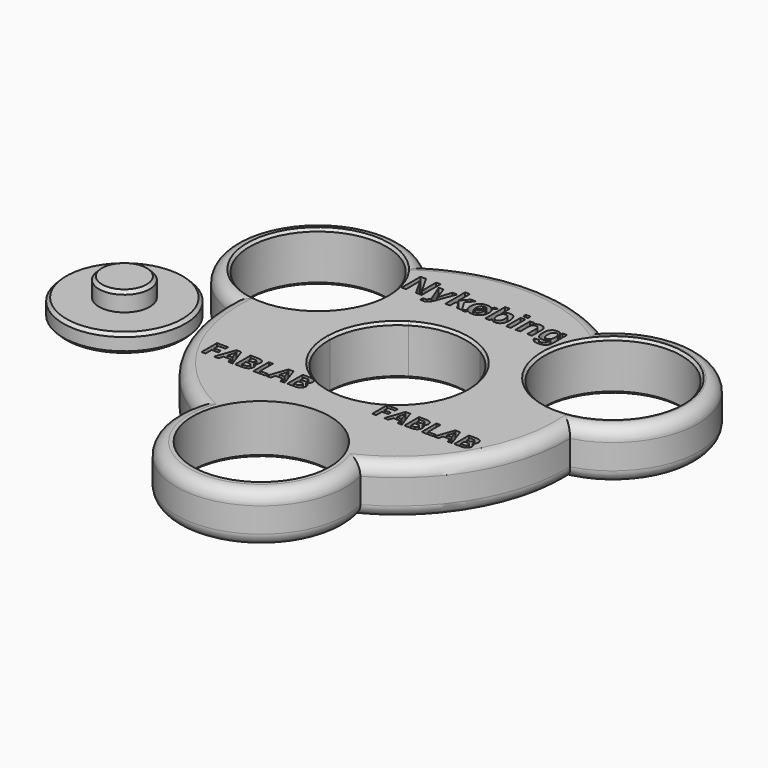
from build123d import *

# Parameters (mm, degrees)
F0_R          = 11
F1_DEPTH      = 8
F2_R          = 2
F3_SIZE       = 0.4
F4_R          = 4.0778592953
F5_DEPTH      = 6
F6_R          = 9.8207891162
F7_DEPTH      = 3
F8_SIZE       = 0.5
F9_SIZE       = 0.5
F10_TEXT_SIZE = 5.4850874186
F11_DEPTH     = 10
F12_TEXT_SIZE = 4.3484511682
F13_TEXT_SIZE = 4.1560128252
F14_DEPTH     = 10


# Not quite as in the source:
# - a feature names something its author has since deleted; it is built from what else it names
# - Text() gives the source's letters only with a copy of the font that has no kerning and outlines rounded to 1/6400 em; it was checked with that copy


with BuildPart() as f1:
    # F0 (on Top) → F1 (new body)
    with BuildSketch(Plane.XY):
        with BuildLine():
            ThreePointArc((-11.0459200084, 0.3002518413), (-9.5695807118, 5.525), (-5.7829857263, 9.4159214148))
            Line((-5.7829857263, 9.4159214148), (-14.3092386636, 23.2984608883))
            ThreePointArc((-14.3092386636, 23.2984608883), (-35.3129874545, 20.3879628128), (-27.3316783301, 0.7429337473))
            Line((-27.3316783301, 0.7429337473), (-11.0459200084, 0.3002518413))
        make_face()
        with Locations((-23.6786706377, 13.6708868667)):
            Circle(F0_R, mode=Mode.SUBTRACT)
        with BuildLine():
            ThreePointArc((5.7000833295, 9.466337731), (9.5695807118, 5.525), (11.0481306206, 0.2032481015))
            Line((11.0481306206, 0.2032481015), (27.3371481996, 0.5029107333))
            ThreePointArc((27.3371481996, 0.5029107333), (35.5144232603, 20.5042618294), (14.1041075707, 23.4232094413))
            Line((14.1041075707, 23.4232094413), (5.7000833295, 9.466337731))
        make_face()
        with Locations((23.6786706377, 13.6708868667)):
            Circle(F0_R, mode=Mode.SUBTRACT)
        with BuildLine():
            Line((13.1991758593, -23.9448188034), (5.3343610648, -9.6771427617))
            ThreePointArc((5.3343610648, -9.6771427617), (0, -11.05), (-5.3343610648, -9.6771427617))
            Line((-5.3343610648, -9.6771427617), (-13.1991758593, -23.9448188034))
            ThreePointArc((-13.1991758593, -23.9448188034), (0, -40.971063743), (13.1991758593, -23.9448188034))
        make_face()
        with Locations((0, -27.3417737335)):
            Circle(F0_R, mode=Mode.SUBTRACT)
        with BuildLine():
            Line((-13.1991758593, -23.9448188034), (-5.3343610648, -9.6771427617))
            ThreePointArc((-5.3343610648, -9.6771427617), (-9.5898645859, -5.4897174085), (-11.0459200084, 0.3002518413))
            Line((-11.0459200084, 0.3002518413), (-27.3316783301, 0.7429337473))
            ThreePointArc((-27.3316783301, 0.7429337473), (-23.72886042, -13.5835847279), (-13.1991758593, -23.9448188034))
        make_face()
        with BuildLine():
            ThreePointArc((-5.7829857263, 9.4159214148), (-0.0485144626, 11.0498934993), (5.7000833295, 9.466337731))
            Line((5.7000833295, 9.466337731), (14.1041075707, 23.4232094413))
            ThreePointArc((14.1041075707, 23.4232094413), (-0.1200426661, 27.3415102116), (-14.3092386636, 23.2984608883))
            Line((-14.3092386636, 23.2984608883), (-5.7829857263, 9.4159214148))
        make_face()
        with BuildLine():
            ThreePointArc((11.0481306206, 0.2032481015), (11.0495326453, 0.1016283491), (11.05, 0))
            ThreePointArc((11.05, 0), (9.5143888339, -5.6195111102), (5.3343610648, -9.6771427617))
            Line((5.3343610648, -9.6771427617), (13.1991758593, -23.9448188034))
            ThreePointArc((13.1991758593, -23.9448188034), (23.6689936822, -13.6876341625), (27.3371481996, 0.5029107333))
            Line((27.3371481996, 0.5029107333), (11.0481306206, 0.2032481015))
        make_face()
    extrude(amount=F1_DEPTH)

    # F2
    f2_edges = [f1.edges().sort_by_distance(p)[0] for p in [
        (-0.120043, 27.34151, 8),
        (-35.312987, 20.387963, 8),
        (-23.72886, -13.583585, 8),
        (0, -40.971064, 8),
        (23.668994, -13.687634, 8),
        (35.514423, 20.504262, 8),
        (23.668994, -13.687634, 0),
        (0, -40.971064, 0),
        (-23.72886, -13.583585, 0),
        (-35.312987, 20.387963, 0),
        (-0.120043, 27.34151, 0),
        (35.514423, 20.504262, 0),
    ]]
    fillet(f2_edges, radius=F2_R)

    # F3
    f3_edges = [f1.edges().sort_by_distance(p)[0] for p in [
        (-11.048131, -0.203248, 8),
        (-34.678671, 13.670887, 8),
        (12.678671, 13.670887, 8),
        (-11, -27.341774, 0),
        (-11.048131, -0.203248, 0),
        (-34.678671, 13.670887, 0),
        (12.678671, 13.670887, 0),
    ]]
    chamfer(f3_edges, length=F3_SIZE)

    # F10 (on Top) → F11 (cut)
    with BuildSketch(Plane.XY):
        with Locations((-12.7465152254, 16.3099450791)):
            Text('Nykøbing', F10_TEXT_SIZE, font='Arimo', font_style=FontStyle.BOLD, text_align=(TextAlign.LEFT, TextAlign.BOTTOM))
    extrude(amount=F11_DEPTH, mode=Mode.SUBTRACT)

    # F12 (on Top) + F13 (on Top) → F14 (cut)
    with BuildSketch(Plane.XY):
        with Locations((-21.4363969862, -13.0258919671)):
            Text('FABLAB', F12_TEXT_SIZE, font='Open Sans', font_style=FontStyle.BOLD, text_align=(TextAlign.LEFT, TextAlign.BOTTOM))
    with BuildSketch(Plane.XY):
        with Locations((5.7687583558, -12.7420239767)):
            Text('FABLAB', F13_TEXT_SIZE, font='Open Sans', font_style=FontStyle.BOLD, text_align=(TextAlign.LEFT, TextAlign.BOTTOM))
    extrude(amount=F14_DEPTH, mode=Mode.SUBTRACT)


with BuildPart() as f5:
    # F4 (on Top) → F5 (new body)
    with BuildSketch(Plane.XY):
        with Locations((-43.8607595861, 0)):
            Circle(F4_R)
    extrude(amount=F5_DEPTH)

    # F6 (on Top) → F7 (join)
    with BuildSketch(Plane.XY):
        with Locations((-43.8607595861, 0)):
            Circle(F6_R)
    extrude(amount=F7_DEPTH)

    # F8
    f8_edges = [f5.edges().sort_by_distance(p)[0] for p in [
        (-47.938619, 0, 6),
    ]]
    chamfer(f8_edges, length=F8_SIZE)

    # F9
    f9_edges = [f5.edges().sort_by_distance(p)[0] for p in [
        (-53.681549, 0, 3),
        (-53.681549, 0, 0),
    ]]
    chamfer(f9_edges, length=F9_SIZE)


solid = Compound([f1.part, f5.part])
